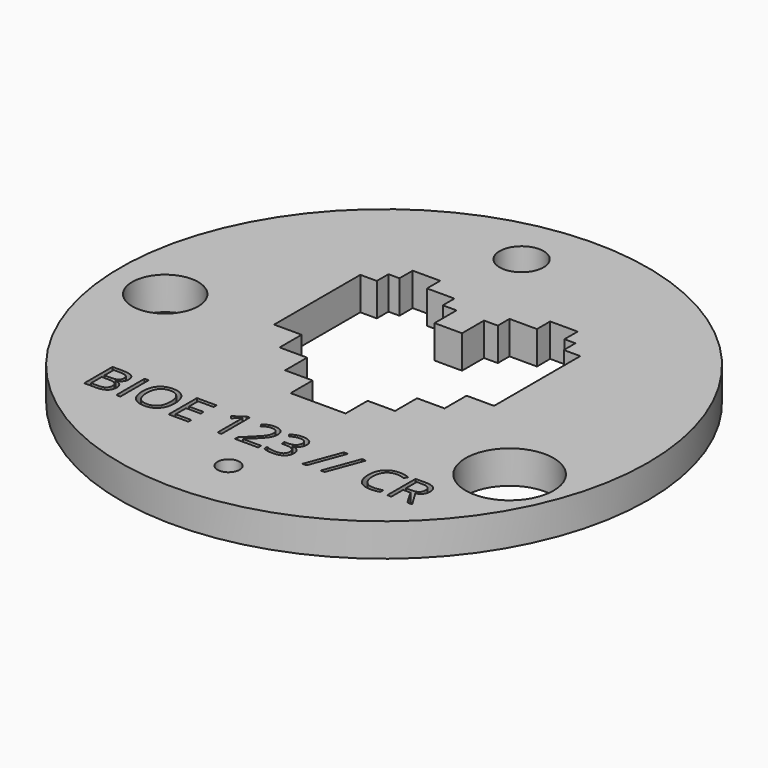
from build123d import *

# Parameters (mm, degrees)
F2_R         = 24
F3_DEPTH     = 3
F4_R         = 3
F4_R_2       = 1
F4_R_3       = 4
F4_R_4       = 2
F5_DEPTH     = 3.001
F7_DEPTH     = 3.001
F8_TEXT_SIZE = 4.5019900426
F9_DEPTH     = 1


# Not quite as in the source:
# - the program builds the solid bodies; features that only make, move or delete a surface that nothing else refers to are left out
# - Text() gives the source's letters only with a copy of the font that has no kerning and outlines rounded to 1/6400 em; it was checked with that copy


with BuildPart() as f3:
    # F2 (on Top) → F3 (new body)
    with BuildSketch(Plane.XY):
        Circle(F2_R)
    extrude(amount=-F3_DEPTH)

    # F4 (on Top) → F5 (cut, through all)
    with BuildSketch(Plane.XY):
        with Locations((-18.9637631246, -1.1728973328)):
            Circle(F4_R)
        with Locations((1.0362368754, -18.9717214068)):
            Circle(F4_R_2)
        with Locations((17.442617518, -7.5335976878)):
            Circle(F4_R_3)
        with Locations((-2.557382482, 18.8271026672)):
            Circle(F4_R_4)
    extrude(amount=-F5_DEPTH, mode=Mode.SUBTRACT)

    # F6 (on Top) → F7 (cut, through all)
    with BuildSketch(Plane.XY):
        Polygon((-2.5, -7.5), (0, -7.5), (2.5, -7.5), (2.5, -5), (5, -5), (5, -2.5), (7.5, -2.5), (7.5, 0), (10, 0), (10, 9.7979589711), (8.5, 9.7979589711), (8.5, 11.1242977306), (7.5, 11.1242977306), (7.5, 12.6242977306), (5, 12.6242977306), (5, 11.1242977306), (2.5, 11.1242977306), (2.5, 9.7979589711), (1.25, 9.7979589711), (1.25, 7.2979589711), (0, 7.2979589711), (-1.25, 7.2979589711), (-1.25, 9.7979589711), (-2.5, 9.7979589711), (-2.5, 11.1242977306), (-5, 11.1242977306), (-5, 12.6242977306), (-7.5, 12.6242977306), (-7.5, 11.1242977306), (-8.5, 11.1242977306), (-8.5, 9.7979589711), (-10, 9.7979589711), (-10, 0), (-7.5, 0), (-7.5, -2.5), (-5, -2.5), (-5, -5), (-2.5, -5), align=None)
    extrude(amount=-F7_DEPTH, mode=Mode.SUBTRACT)

    # F8 (on Top) → F9 (cut)
    with BuildSketch(Plane.XY):
        with Locations((-15.3417356487, -15.4594117776)):
            Text('BIOE 123 // CR', F8_TEXT_SIZE, font='Open Sans', text_align=(TextAlign.LEFT, TextAlign.BOTTOM))
    extrude(amount=-F9_DEPTH, mode=Mode.SUBTRACT)


solid = f3.part
